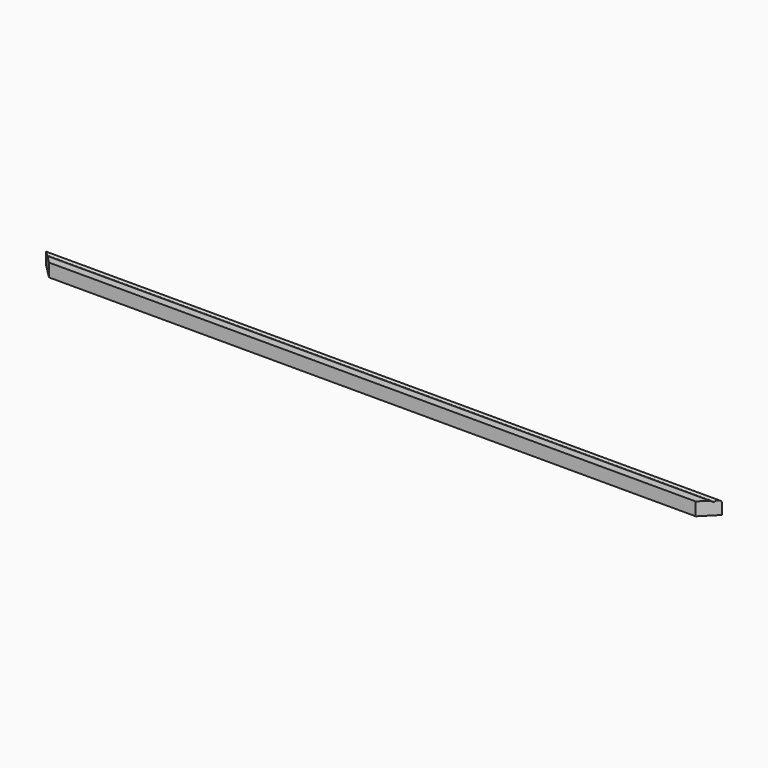
from build123d import *

# Parameters (mm, degrees)
F1_DEPTH = 736.6
F2_SIZE  = 31.74999


# Not quite as in the source:
# - a fillet or chamfer is up to 0.001 mm smaller than in the source, because OpenCascade refuses the exact size


with BuildPart() as f1:
    # F0 (on Right) → F1 (new body, symmetric)
    with BuildSketch(Plane.YZ):
        with BuildLine():
            Line((-15.875, -14.2875), (15.875, -14.2875))
            Line((15.875, -14.2875), (15.875, 9.525))
            ThreePointArc((15.875, 9.525), (12.4385421004, 14.0991686237), (7.08843051, 12.07220847))
            ThreePointArc((7.08843051, 12.07220847), (5.9853917743, 11.4055483551), (4.789455264, 11.886033552))
            ThreePointArc((4.789455264, 11.886033552), (2.3755826554, 13.6595328458), (-0.5531949, 14.2875))
            Line((-0.5531949, 14.2875), (-15.875, 14.2875))
            Line((-15.875, 14.2875), (-15.875, -14.2875))
        make_face()
    extrude(amount=F1_DEPTH, both=True)

    # F2 (size 31.75 in the source; OpenCascade refuses exactly that, so slightly less here)
    f2_edges = [f1.edges().sort_by_distance(p)[0] for p in [
        (-736.6, -15.875, 0),
        (736.6, -15.875, 0),
    ]]
    chamfer(f2_edges, length=F2_SIZE)


solid = f1.part
